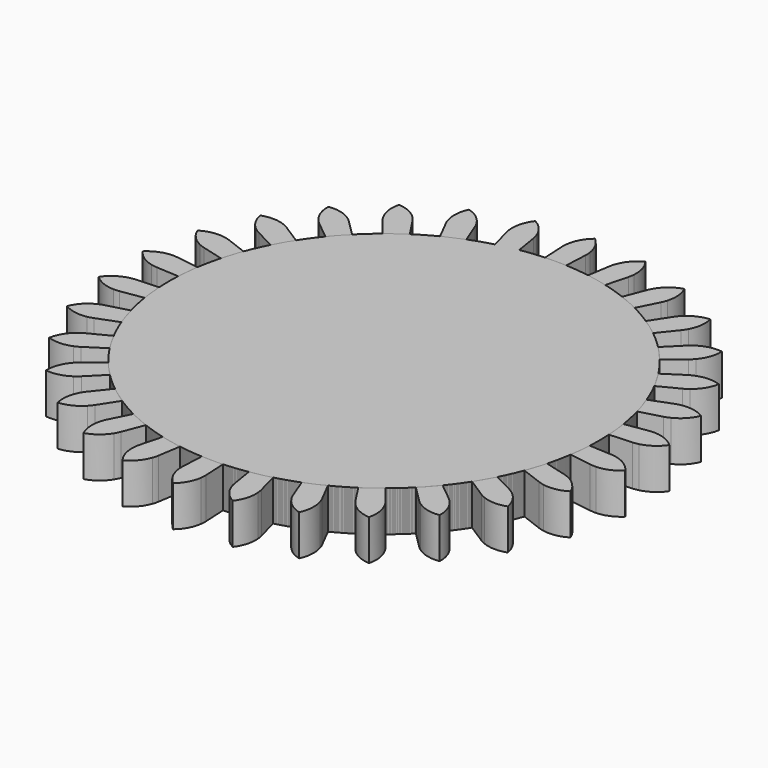
from build123d import *

# Parameters (mm, degrees)
F1_DEPTH = 0.5
F2_COUNT = 30


with BuildPart() as f1:
    # F0 (on Top) → F1 (new body)
    with BuildSketch(Plane.XY):
        with BuildLine():
            ThreePointArc((-0.1354396104, 2.6465366258), (-1.8253198394, -1.9211214131), (2.65, 0))
            ThreePointArc((2.65, 0), (2.2496901091, 1.4004979161), (1.1697023299, 2.3778764601))
            ThreePointArc((1.1697023299, 2.3778764601), (1.0512580514, 2.4325617175), (0.9302659747, 2.4813514899))
            ThreePointArc((0.9302659747, 2.4813514899), (0.5342933786, 2.5955790463), (0.1253986636, 2.6470313892))
            ThreePointArc((0.1253986636, 2.6470313892), (0.060204291, 2.6493160331), (-0.0050265645, 2.6499952328))
            ThreePointArc((-0.0050265645, 2.6499952328), (-0.070254374, 2.6490685765), (-0.1354396104, 2.6465366258))
        make_face()
        with BuildLine():
            Line((-0.0056904504, 2.9999946031), (-0.0050265645, 2.6499952328))
            ThreePointArc((-0.0050265645, 2.6499952328), (0.060204291, 2.6493160331), (0.1253986636, 2.6470313892))
            Line((0.1253986636, 2.6470313892), (0.1384951147, 2.9234834352))
            ThreePointArc((0.1384951147, 2.9234834352), (0.1385702752, 2.9602871406), (0.1353155846, 2.9969467284))
            ThreePointArc((0.1353155846, 2.9969467284), (0.0648304808, 2.9992994197), (-0.0056904504, 2.9999946031))
        make_face()
        with BuildLine():
            ThreePointArc((-0.1466839081, 2.996411826), (-0.0762082368, 2.9990318946), (-0.0056904504, 2.9999946031))
            Line((-0.0056904504, 2.9999946031), (-0.0061722418, 3.2539941462))
            ThreePointArc((-0.0061722418, 3.2539941462), (-0.1004855069, 3.1383263629), (-0.1466839081, 2.996411826))
        make_face()
        with BuildLine():
            Line((-0.0061722418, 3.2539941462), (-0.0056904504, 2.9999946031))
            ThreePointArc((-0.0056904504, 2.9999946031), (0.0648304808, 2.9992994197), (0.1353155846, 2.9969467284))
            ThreePointArc((0.1353155846, 2.9969467284), (0.088579145, 3.1386849846), (-0.0061722418, 3.2539941462))
        make_face()
        with BuildLine():
            Line((-0.1495847231, 2.9229369995), (-0.1354396104, 2.6465366258))
            ThreePointArc((-0.1354396104, 2.6465366258), (-0.070254374, 2.6490685765), (-0.0050265645, 2.6499952328))
            Line((-0.0050265645, 2.6499952328), (-0.0056904504, 2.9999946031))
            ThreePointArc((-0.0056904504, 2.9999946031), (-0.0762082368, 2.9990318946), (-0.1466839081, 2.996411826))
            ThreePointArc((-0.1466839081, 2.996411826), (-0.1497995026, 2.959740155), (-0.1495847231, 2.9229369995))
        make_face()
    extrude(amount=F1_DEPTH)


with BuildPart() as f2_1:
    # F2: instance of F1
    add(f1.part.rotate(Axis((0, 0, 0), (0, 0, -1)), 1 * 360 / F2_COUNT))


with BuildPart() as f2_2:
    # F2: instance of F1
    add(f1.part.rotate(Axis((0, 0, 0), (0, 0, -1)), 2 * 360 / F2_COUNT))


with BuildPart() as f2_3:
    # F2: instance of F1
    add(f1.part.rotate(Axis((0, 0, 0), (0, 0, -1)), 3 * 360 / F2_COUNT))


with BuildPart() as f2_4:
    # F2: instance of F1
    add(f1.part.rotate(Axis((0, 0, 0), (0, 0, -1)), 4 * 360 / F2_COUNT))


with BuildPart() as f2_5:
    # F2: instance of F1
    add(f1.part.rotate(Axis((0, 0, 0), (0, 0, -1)), 5 * 360 / F2_COUNT))


with BuildPart() as f2_6:
    # F2: instance of F1
    add(f1.part.rotate(Axis((0, 0, 0), (0, 0, -1)), 6 * 360 / F2_COUNT))


with BuildPart() as f2_7:
    # F2: instance of F1
    add(f1.part.rotate(Axis((0, 0, 0), (0, 0, -1)), 7 * 360 / F2_COUNT))


with BuildPart() as f2_8:
    # F2: instance of F1
    add(f1.part.rotate(Axis((0, 0, 0), (0, 0, -1)), 8 * 360 / F2_COUNT))


with BuildPart() as f2_9:
    # F2: instance of F1
    add(f1.part.rotate(Axis((0, 0, 0), (0, 0, -1)), 9 * 360 / F2_COUNT))


with BuildPart() as f2_10:
    # F2: instance of F1
    add(f1.part.rotate(Axis((0, 0, 0), (0, 0, -1)), 10 * 360 / F2_COUNT))


with BuildPart() as f2_11:
    # F2: instance of F1
    add(f1.part.rotate(Axis((0, 0, 0), (0, 0, -1)), 11 * 360 / F2_COUNT))


with BuildPart() as f2_12:
    # F2: instance of F1
    add(f1.part.rotate(Axis((0, 0, 0), (0, 0, -1)), 12 * 360 / F2_COUNT))


with BuildPart() as f2_13:
    # F2: instance of F1
    add(f1.part.rotate(Axis((0, 0, 0), (0, 0, -1)), 13 * 360 / F2_COUNT))


with BuildPart() as f2_14:
    # F2: instance of F1
    add(f1.part.rotate(Axis((0, 0, 0), (0, 0, -1)), 14 * 360 / F2_COUNT))


with BuildPart() as f2_15:
    # F2: instance of F1
    add(f1.part.rotate(Axis((0, 0, 0), (0, 0, -1)), 15 * 360 / F2_COUNT))


with BuildPart() as f2_16:
    # F2: instance of F1
    add(f1.part.rotate(Axis((0, 0, 0), (0, 0, -1)), 16 * 360 / F2_COUNT))


with BuildPart() as f2_17:
    # F2: instance of F1
    add(f1.part.rotate(Axis((0, 0, 0), (0, 0, -1)), 17 * 360 / F2_COUNT))


with BuildPart() as f2_18:
    # F2: instance of F1
    add(f1.part.rotate(Axis((0, 0, 0), (0, 0, -1)), 18 * 360 / F2_COUNT))


with BuildPart() as f2_19:
    # F2: instance of F1
    add(f1.part.rotate(Axis((0, 0, 0), (0, 0, -1)), 19 * 360 / F2_COUNT))


with BuildPart() as f2_20:
    # F2: instance of F1
    add(f1.part.rotate(Axis((0, 0, 0), (0, 0, -1)), 20 * 360 / F2_COUNT))


with BuildPart() as f2_21:
    # F2: instance of F1
    add(f1.part.rotate(Axis((0, 0, 0), (0, 0, -1)), 21 * 360 / F2_COUNT))


with BuildPart() as f2_22:
    # F2: instance of F1
    add(f1.part.rotate(Axis((0, 0, 0), (0, 0, -1)), 22 * 360 / F2_COUNT))


with BuildPart() as f2_23:
    # F2: instance of F1
    add(f1.part.rotate(Axis((0, 0, 0), (0, 0, -1)), 23 * 360 / F2_COUNT))


with BuildPart() as f2_24:
    # F2: instance of F1
    add(f1.part.rotate(Axis((0, 0, 0), (0, 0, -1)), 24 * 360 / F2_COUNT))


with BuildPart() as f2_25:
    # F2: instance of F1
    add(f1.part.rotate(Axis((0, 0, 0), (0, 0, -1)), 25 * 360 / F2_COUNT))


with BuildPart() as f2_26:
    # F2: instance of F1
    add(f1.part.rotate(Axis((0, 0, 0), (0, 0, -1)), 26 * 360 / F2_COUNT))


with BuildPart() as f2_27:
    # F2: instance of F1
    add(f1.part.rotate(Axis((0, 0, 0), (0, 0, -1)), 27 * 360 / F2_COUNT))


with BuildPart() as f2_28:
    # F2: instance of F1
    add(f1.part.rotate(Axis((0, 0, 0), (0, 0, -1)), 28 * 360 / F2_COUNT))


with BuildPart() as f2_29:
    # F2: instance of F1
    add(f1.part.rotate(Axis((0, 0, 0), (0, 0, -1)), 29 * 360 / F2_COUNT))


solid = Compound([f1.part, f2_1.part, f2_2.part, f2_3.part, f2_4.part, f2_5.part, f2_6.part, f2_7.part, f2_8.part, f2_9.part, f2_10.part, f2_11.part, f2_12.part, f2_13.part, f2_14.part, f2_15.part, f2_16.part, f2_17.part, f2_18.part, f2_19.part, f2_20.part, f2_21.part, f2_22.part, f2_23.part, f2_24.part, f2_25.part, f2_26.part, f2_27.part, f2_28.part, f2_29.part])
